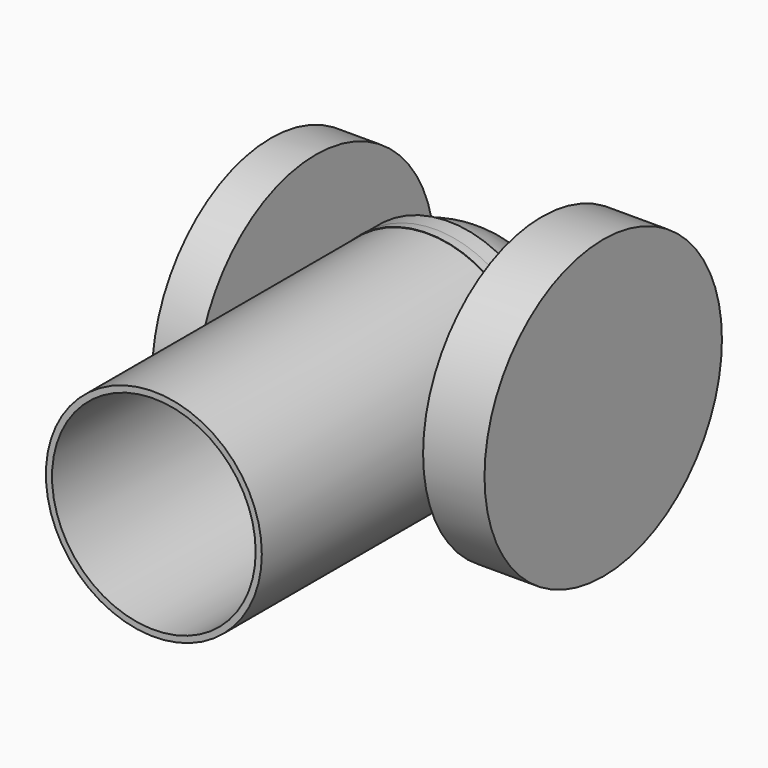
from build123d import *

# Parameters (mm, degrees)
F0_R      = 44.6495362372
F1_DEPTH  = 76.2
F2_R      = 44.6495362372
F3_DEPTH  = 25.4
F4_T      = -2.54
F7_R      = 42.1640685754
F8_DEPTH  = 35.814
F11_T     = 2.54
F12_DEPTH = 39.878
F13_DEPTH = 152.4
F15_R     = 61.4381717254
F16_DEPTH = 18.542
F18_R     = 61.3590086079
F19_DEPTH = 25.4


# Not quite as in the source:
# - a feature of the source that left no trace in its solid (it failed there, or was rolled back) is left out
# - a shell that OpenCascade refuses in one call is made with other operations: the cavity is built on its own and cut out


with BuildPart() as f1:
    # F0 (on Front) → F1 (new body)
    with BuildSketch(Plane.XZ):
        Circle(F0_R)
    extrude(amount=F1_DEPTH)

    # F2 (on face) → F3 (join)
    with BuildSketch(Plane.XZ.offset(76.2)):
        Circle(F2_R)
    extrude(amount=F3_DEPTH)

    # F4
    f4_openings = [f1.faces().sort_by_distance(p)[0] for p in [
        (0, -101.6, 0),
    ]]
    offset(amount=F4_T, openings=f4_openings)

    # F5 (on Top) → F6 (revolve)
    with BuildSketch(Plane.XY):
        with BuildLine():
            Line((0, 0), (44.8180213571, 0))
            ThreePointArc((44.8180213571, 0), (31.7807876043, 32.2353759655), (0, 46.3446093542))
            Line((0, 46.3446093542), (0, 0))
        make_face()
    revolve(axis=Axis((0, 23.1723046771, 0), (0, -1, 0)))

    # F7 (on face) → F8 (join)
    with BuildSketch(Plane.XZ.offset(2.54)):
        Circle(F7_R)
    extrude(amount=F8_DEPTH)

    # F11: shell of thickness 2.54, made by hand


with BuildPart() as f10:
    # F9 (on Front) → F10 (revolve)
    with BuildSketch(Plane.XZ):
        with BuildLine():
            ThreePointArc((0, -41.6139443904), (29.4255022704, -29.4255022704), (41.6139443904, 0))
            ThreePointArc((41.6139443904, 0), (29.4255022704, 29.4255022704), (0, 41.6139443904))
            Line((0, 41.6139443904), (0, -41.6139443904))
        make_face()
    revolve(axis=Axis((0, 0, 0), (0, 0, 1)))


with BuildPart() as f11_core1:
    # F11_t2: copy of F1
    add(f1.part)

    # the walls: a layer under each face that stays
    f11_faces = [f11_core1.faces().sort_by_distance(p)[0] for p in [
        (-39.2157686874, 0, -21.5790473201),
        (-31.7807876043, 32.2353759655, 0),
        (-44.6495362372, -50.8, 0),
        (-41.672900488, -101.6, -11.9065429966),
        (-42.1095362372, -69.977, 0),
    ]]
    thicken(f11_faces, amount=-F11_T, mode=Mode.SUBTRACT)

    # F11_s3 → F11_t4 (revolve, cut)
    with BuildSketch(Plane.XY):
        Polygon((44.6749362372, -0.0254), (44.6495362372, 2.54), (42.1095362372, 2.54), (42.1095362372, 0), align=None)
    revolve(axis=Axis((0, 0, 0), (0, -1, 0)), mode=Mode.SUBTRACT)


with BuildPart() as f1_1:
    add(f1.part)

    # what is left inside the walls is the cavity
    f11_cavity = [f11_core1.part.solids().sort_by_distance(p)[0] for p in [
        (-35.782256, 22.913005, 0),
    ]]
    add(f11_cavity, mode=Mode.SUBTRACT)

    # F12 (add): a face of the model
    f12_faces = [f1_1.faces().sort_by_distance(p)[0] for p in [
        (-43.3866566432, -101.6, 0),
    ]]
    extrude(f12_faces, amount=F12_DEPTH)

    # F13 (add): a face of the model
    f13_faces = [f1_1.faces().sort_by_distance(p)[0] for p in [
        (-43.3866566432, -141.478, 0),
    ]]
    extrude(f13_faces, amount=-F13_DEPTH)


with BuildPart() as f16:
    # F15 (on offset) → F16 (new body)
    with BuildSketch(Plane.YZ.offset(-46.228)):
        with Locations((0, -3.0824954156)):
            Circle(F15_R)
    extrude(amount=-F16_DEPTH)


with BuildPart() as f19:
    # F18 (on offset) → F19 (new body)
    with BuildSketch(Plane.YZ.offset(45.212)):
        with Locations((2.5428049266, 3.0883017462)):
            Circle(F18_R)
    extrude(amount=F19_DEPTH)


solid = Compound([f10.part, f1_1.part, f16.part, f19.part])
